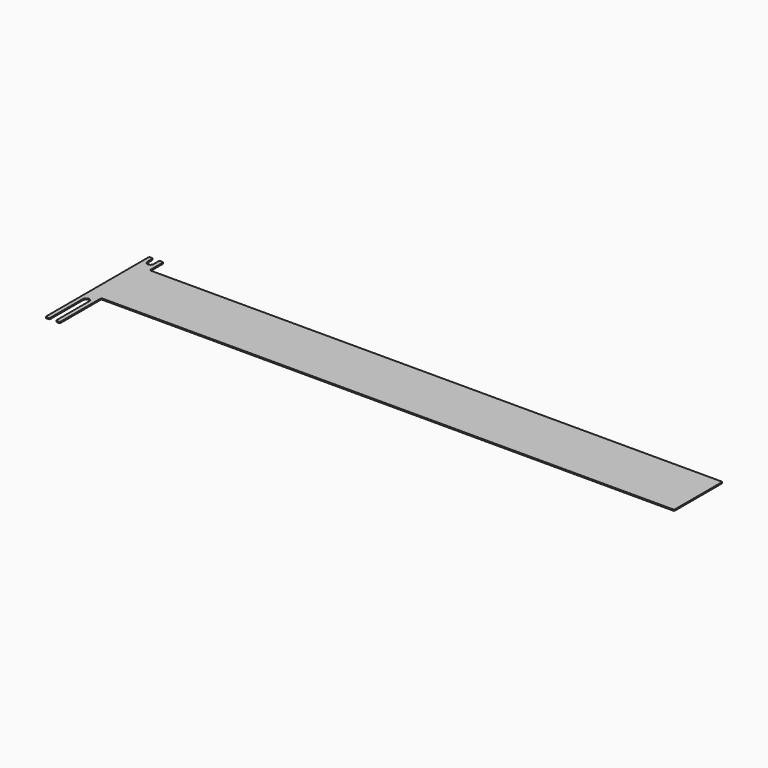
from build123d import *

# Parameters (mm, degrees)
F0_W     = 1020
F0_H     = 105
F1_DEPTH = 2
F3_DEPTH = 2
F6_W     = 69.2964494228
F6_H     = 80
F7_DEPTH = 2.001
F8_R     = 5.44999
F9_R     = 2


# Not quite as in the source:
# - a fillet or chamfer is up to 0.001 mm smaller than in the source, because OpenCascade refuses the exact size


with BuildPart() as f1:
    # F0 (on Top) → F1 (new body)
    with BuildSketch(Plane.XY):
        Rectangle(F0_W, F0_H)
    extrude(amount=F1_DEPTH)

    # F2 (on face) → F3 (join)
    with BuildSketch(Plane.XY.offset(2)):
        Polygon((-485, -52.5), (-510, -52.5), (-510, -142.5), (-503, -142.5), (-503, -64.5), (-492.1, -64.5), (-492.1, -142.5), (-485, -142.5), align=None)
    extrude(amount=-F3_DEPTH)

    # F5: F1 across plane


with BuildPart() as f1_1:
    add(f1.part)
    add(f1.part.mirror(Plane.XZ))

    # F6 (on face) → F7 (cut, through all)
    with BuildSketch(Plane.XY.offset(2)):
        with Locations((-500.6258040667, 122.5)):
            Rectangle(F6_W, F6_H)
    extrude(amount=-F7_DEPTH, mode=Mode.SUBTRACT)

    # F8 (radius 5.45 in the source; OpenCascade refuses exactly that, so slightly less here)
    f8_edges = [f1_1.edges().sort_by_distance(p)[0] for p in [
        (-503, -64.5, 1),
        (-492.1, -64.5, 1),
        (-503, 64.5, 1),
        (-492.1, 64.5, 1),
    ]]
    fillet(f8_edges, radius=F8_R)

    # F9
    f9_edges = [f1_1.edges().sort_by_distance(p)[0] for p in [
        (-485, 52.5, 1),
        (-485, 82.5, 1),
        (-492.1, 82.5, 1),
        (-503, 82.5, 1),
        (-510, 82.5, 1),
        (-485, -52.5, 1),
        (-485, -142.5, 1),
        (-492.1, -142.5, 1),
        (-503, -142.5, 1),
        (-510, -142.5, 1),
        (510, -52.5, 1),
        (510, 52.5, 1),
    ]]
    fillet(f9_edges, radius=F9_R)


solid = f1_1.part
